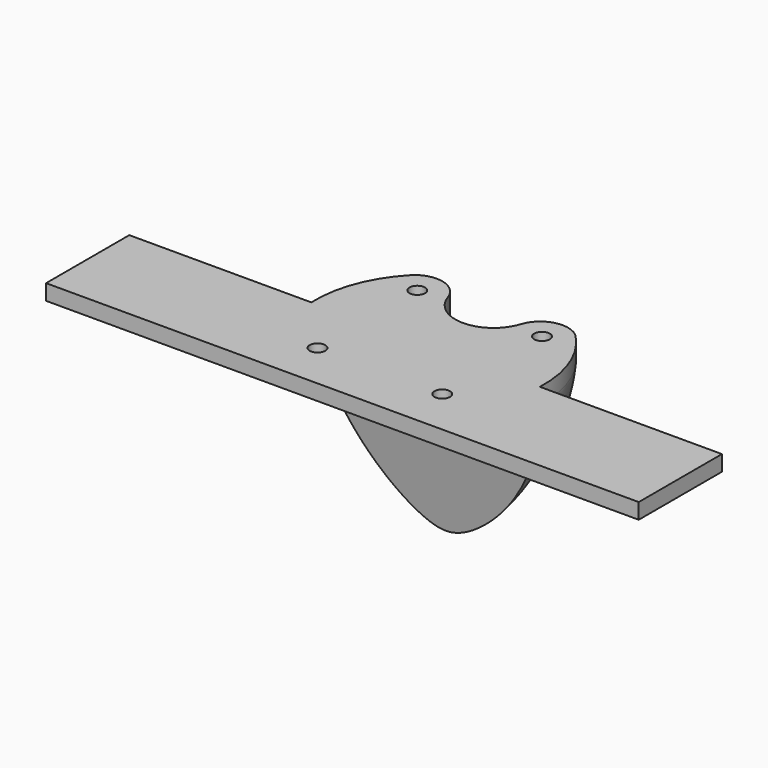
from build123d import *

# Parameters (mm, degrees)
F0_R     = 1.5
F1_DEPTH = 3
F5_DEPTH = 25
F7_DEPTH = 35


# Not quite as in the source:
# - a feature names something its author has since deleted; it is built from what else it names


with BuildPart() as f1:
    # F0 (on Top) → F1 (new body)
    with BuildSketch(Plane.XY):
        with BuildLine():
            Line((6.5574385243, -21), (57, -21))
            Line((57, -21), (57, -1))
            Line((57, -1), (21.9772609758, -1))
            ThreePointArc((21.9772609758, -1), (0, 22), (-21.9772609758, -1))
            Line((-21.9772609758, -1), (-57, -1))
            Line((-57, -1), (-57, -21))
            Line((-57, -21), (6.5574385243, -21))
        make_face()
        with Locations((-12, -12)):
            Circle(F0_R, mode=Mode.SUBTRACT)
        with Locations((12, -12)):
            Circle(F0_R, mode=Mode.SUBTRACT)
        with Locations((-12, 12)):
            Circle(F0_R, mode=Mode.SUBTRACT)
        with Locations((12, 12)):
            Circle(F0_R, mode=Mode.SUBTRACT)
    extrude(amount=F1_DEPTH)

    # F2 (on Right) → F3 (revolve)
    with BuildSketch(Plane.YZ):
        with BuildLine():
            Line((0, 0), (0, -32.8796606992))
            ThreePointArc((0, -32.8796606992), (15.0334447446, -19.1386350968), (22, 0))
            Line((22, 0), (0, 0))
        make_face()
    revolve(axis=Axis((0, 0, -16.4398303496), (0, 0, -1)))

    # F4 (on Right) → F5 (cut, symmetric)
    with BuildSketch(Plane.YZ):
        Polygon((7.20365692, -51.6230810942), (-0.9809204616, 0.0523067461), (-22.7521642769, 0), (-21.7191129923, -52.1955192089), align=None)
    extrude(amount=F5_DEPTH, both=True, mode=Mode.SUBTRACT)

    # F6 (on face) → F7 (cut)
    with BuildSketch(Plane.XY.offset(3)):
        with BuildLine():
            ThreePointArc((-15.7890972634, 15.3200655223), (-10.8662470151, 16.6578455627), (-7.0613301317, 13.2597994308))
            ThreePointArc((-7.0613301317, 13.2597994308), (0, 8.0029264883), (7.0613301317, 13.2597994308))
            ThreePointArc((7.0613301317, 13.2597994308), (10.8662470151, 16.6578455627), (15.7890972634, 15.3200655223))
            ThreePointArc((15.7890972634, 15.3200655223), (0, 22), (-15.7890972634, 15.3200655223))
        make_face()
    extrude(amount=-F7_DEPTH, mode=Mode.SUBTRACT)


solid = f1.part
